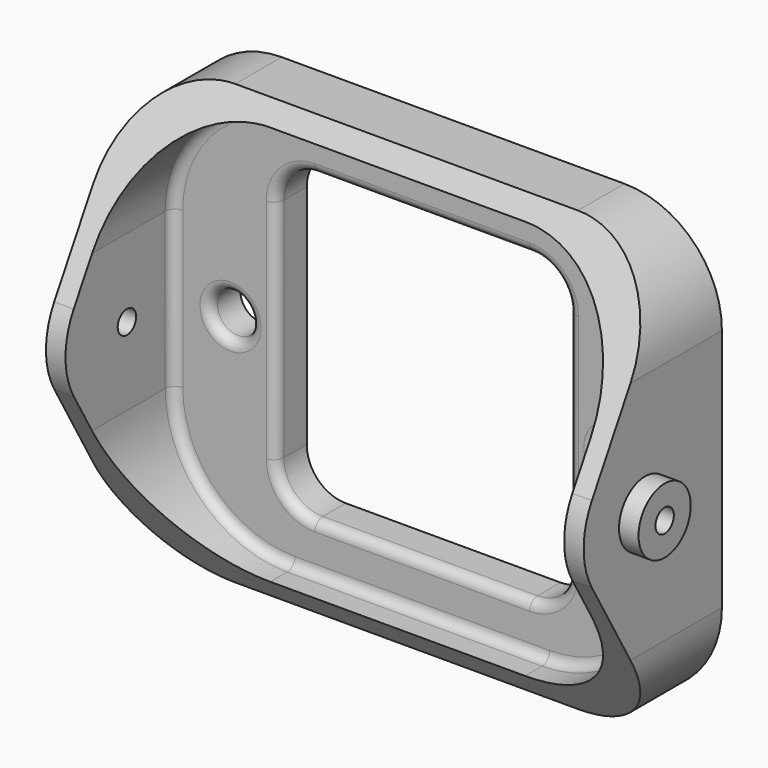
from build123d import *
from build123d import SkipClean  # not in build123d's __all__

# Parameters (mm, degrees)
F0_R           = 1.0795
F1_DEPTH       = 2
F3_DEPTH       = 19.9898
F4_R           = 0.508
F5_R           = 0.6
F6_DEPTH       = 28.0045
F7_R           = 1.7
F7_R_2         = 0.6
F8_DEPTH       = 1.016
F9_R           = 1.7
F9_R_2         = 0.6
F10_DEPTH      = 1.016
F12_DEPTH      = 25.4
F12_DEPTH_BACK = 25.4


# Not quite as in the source:
# - after a boolean that leaves OpenCascade's solid faulty, fix() repairs it


with BuildPart() as f1:
    # F0 (on Front) → F1 (new body)
    with BuildSketch(Plane.XZ):
        with BuildLine():
            Line((8.92175, 11.43), (-8.92175, 11.43))
            ThreePointArc((-8.92175, 11.43), (-12.5138524484, 9.9421024484), (-14.00175, 6.35))
            Line((-14.00175, 6.35), (-14.00175, -6.35))
            ThreePointArc((-14.00175, -6.35), (-12.5138524484, -9.9421024484), (-8.92175, -11.43))
            Line((-8.92175, -11.43), (8.92175, -11.43))
            ThreePointArc((8.92175, -11.43), (12.5138524484, -9.9421024484), (14.00175, -6.35))
            Line((14.00175, -6.35), (14.00175, 6.35))
            ThreePointArc((14.00175, 6.35), (12.5138524484, 9.9421024484), (8.92175, 11.43))
        make_face()
        with Locations((-9.9949, 0)):
            Circle(F0_R, mode=Mode.SUBTRACT)
        with BuildLine():
            ThreePointArc((-7.62, 5.9055), (-7.0248409794, 7.3423409794), (-5.588, 7.9375))
            Line((-5.588, 7.9375), (5.588, 7.9375))
            ThreePointArc((5.588, 7.9375), (7.0248409794, 7.3423409794), (7.62, 5.9055))
            Line((7.62, 5.9055), (7.62, -5.9055))
            ThreePointArc((7.62, -5.9055), (7.0248409794, -7.3423409794), (5.588, -7.9375))
            Line((5.588, -7.9375), (-5.588, -7.9375))
            ThreePointArc((-5.588, -7.9375), (-7.0248409794, -7.3423409794), (-7.62, -5.9055))
            Line((-7.62, -5.9055), (-7.62, 5.9055))
        make_face(mode=Mode.SUBTRACT)
        with Locations((9.9949, 0)):
            Circle(F0_R, mode=Mode.SUBTRACT)
    extrude(amount=F1_DEPTH)

    # F2 (on face) → F3 (join)
    with BuildSketch(Plane.XZ.offset(2)):
        with BuildLine():
            Line((8.92175, 11.43), (-8.92175, 11.43))
            ThreePointArc((-8.92175, 11.43), (-12.5138524484, 9.9421024484), (-14.00175, 6.35))
            Line((-14.00175, 6.35), (-14.00175, -6.35))
            ThreePointArc((-14.00175, -6.35), (-12.5138524484, -9.9421024484), (-8.92175, -11.43))
            Line((-8.92175, -11.43), (8.92175, -11.43))
            ThreePointArc((8.92175, -11.43), (12.5138524484, -9.9421024484), (14.00175, -6.35))
            Line((14.00175, -6.35), (14.00175, 6.35))
            ThreePointArc((14.00175, 6.35), (12.5138524484, 9.9421024484), (8.92175, 11.43))
        make_face()
        with BuildLine():
            ThreePointArc((-12.98575, 4.064), (-11.1258780605, 8.5541280605), (-6.63575, 10.414))
            Line((-6.63575, 10.414), (6.63575, 10.414))
            ThreePointArc((6.63575, 10.414), (11.1258780605, 8.5541280605), (12.98575, 4.064))
            Line((12.98575, 4.064), (12.98575, -4.064))
            ThreePointArc((12.98575, -4.064), (11.1258780605, -8.5541280605), (6.63575, -10.414))
            Line((6.63575, -10.414), (-6.63575, -10.414))
            ThreePointArc((-6.63575, -10.414), (-11.1258780605, -8.5541280605), (-12.98575, -4.064))
            Line((-12.98575, -4.064), (-12.98575, 4.064))
        make_face(mode=Mode.SUBTRACT)
    extrude(amount=F3_DEPTH)

    # F4
    f4_edges = [f1.edges().sort_by_distance(p)[0] for p in [
        (-11.125878, -2, -8.554128),
        (-12.98575, -2, 0),
        (-11.125878, -2, 8.554128),
        (0, -2, 10.414),
        (11.125878, -2, 8.554128),
        (12.98575, -2, 0),
        (11.125878, -2, -8.554128),
        (0, -2, -10.414),
        (-11.0744, -2, 0),
        (-7.62, -2, 0),
        (-7.024841, -2, -7.342341),
        (-7.024841, -2, 7.342341),
        (0, -2, -7.9375),
        (0, -2, 7.9375),
        (7.024841, -2, -7.342341),
        (7.024841, -2, 7.342341),
        (7.62, -2, 0),
        (8.9154, -2, 0),
    ]]
    fillet(f4_edges, radius=F4_R)

    # F5 (on face) → F6 (cut, through all)
    with BuildSketch(Plane.YZ.offset(14.00175)):
        with Locations((-5, 0)):
            Circle(F5_R)
        with Locations((-11, 0)):
            Circle(F5_R)
    extrude(amount=-F6_DEPTH, mode=Mode.SUBTRACT)

    # F7 (on face) → F8 (join)
    with BuildSketch(Plane.YZ.offset(14.00175)):
        with Locations((-5, 0)):
            Circle(F7_R)
        with Locations((-5, 0)):
            Circle(F7_R_2, mode=Mode.SUBTRACT)
        with Locations((-11, 0)):
            Circle(F7_R)
        with Locations((-11, 0)):
            Circle(F7_R_2, mode=Mode.SUBTRACT)
    extrude(amount=F8_DEPTH)

    # F9 (on face) → F10 (join)
    with BuildSketch(Plane(origin=(-14.00175, 0, 0), x_dir=(0, -1, 0), z_dir=(-1, 0, 0))):
        with Locations((11, 0)):
            Circle(F9_R)
        with Locations((11, 0)):
            Circle(F9_R_2, mode=Mode.SUBTRACT)
        with Locations((5, 0)):
            Circle(F9_R)
        with Locations((5, 0)):
            Circle(F9_R_2, mode=Mode.SUBTRACT)
    with SkipClean():  # cleaning this boolean's faces spoils the solid; the shape is the same uncleaned
        extrude(amount=F10_DEPTH)

    # F11 (on Right) → F12 (cut, two sides)
    with BuildSketch(Plane.YZ) as f12_sk:
        with BuildLine():
            ThreePointArc((-8.4645346278, -2.00025), (-9.0005, 0), (-8.4645346278, 2.00025))
            Line((-8.4645346278, 2.00025), (-2.2869158186, 12.7001996474))
            Line((-2.2869158186, 12.7001996474), (-49.9461684498, 19.8914812337))
            Line((-49.9461684498, 19.8914812337), (-49.9461684498, -23.9422454613))
            Line((-49.9461684498, -23.9422454613), (4.2036823583, -23.9422454613))
            Line((4.2036823583, -23.9422454613), (-8.4645346278, -2.00025))
        make_face()
    extrude(amount=-F12_DEPTH, mode=Mode.SUBTRACT)
    extrude(f12_sk.sketch, amount=F12_DEPTH_BACK, mode=Mode.SUBTRACT)

    add(f1.part.fix(), mode=Mode.REPLACE)


solid = f1.part
